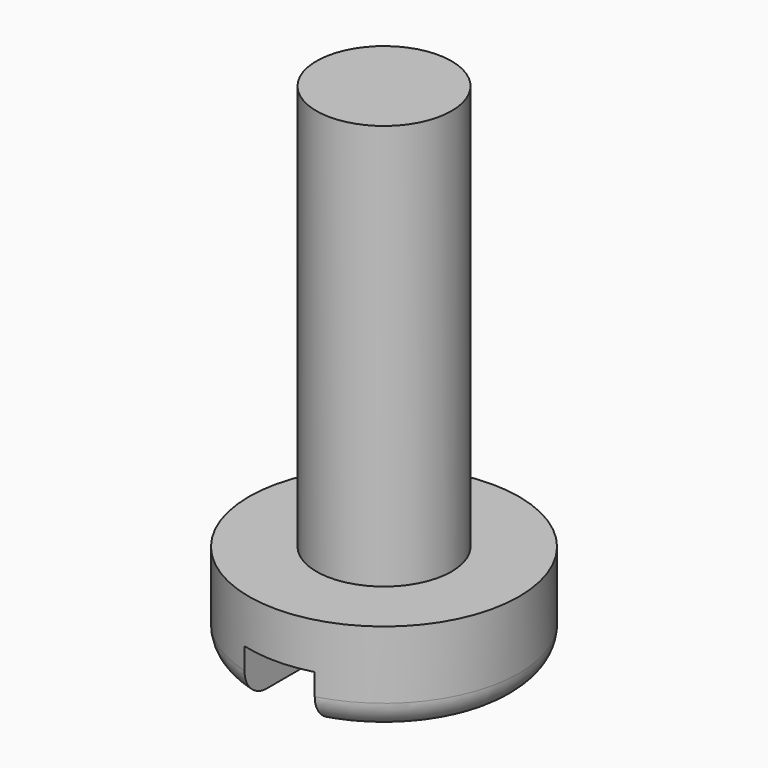
from build123d import *

# Parameters (mm, degrees)
F0_R     = 3.175
F1_DEPTH = 19.05
F2_R     = 6.35
F3_DEPTH = 4.445
F4_W     = 3.302
F4_H     = 26.5450086477
F5_DEPTH = 2.286
F6_R     = 1.27


with BuildPart() as f1:
    # F0 (on Top) → F1 (new body)
    with BuildSketch(Plane.XY):
        Circle(F0_R)
    extrude(amount=F1_DEPTH)

    # F2 (on face) → F3 (join)
    with BuildSketch(Plane(origin=(0, 0, 0), x_dir=(1, 0, 0), z_dir=(0, 0, -1))):
        Circle(F2_R)
    extrude(amount=F3_DEPTH)

    # F4 (on face) → F5 (cut)
    with BuildSketch(Plane(origin=(0, 0, -4.445), x_dir=(1, 0, 0), z_dir=(0, 0, -1))):
        Rectangle(F4_W, F4_H)
    extrude(amount=-F5_DEPTH, mode=Mode.SUBTRACT)

    # F6
    f6_edges = [f1.edges().sort_by_distance(p)[0] for p in [
        (-6.35, 0, -4.445),
        (5.040156, 3.862554, -4.445),
        (5.040156, -3.862554, -4.445),
    ]]
    fillet(f6_edges, radius=F6_R)


solid = f1.part
